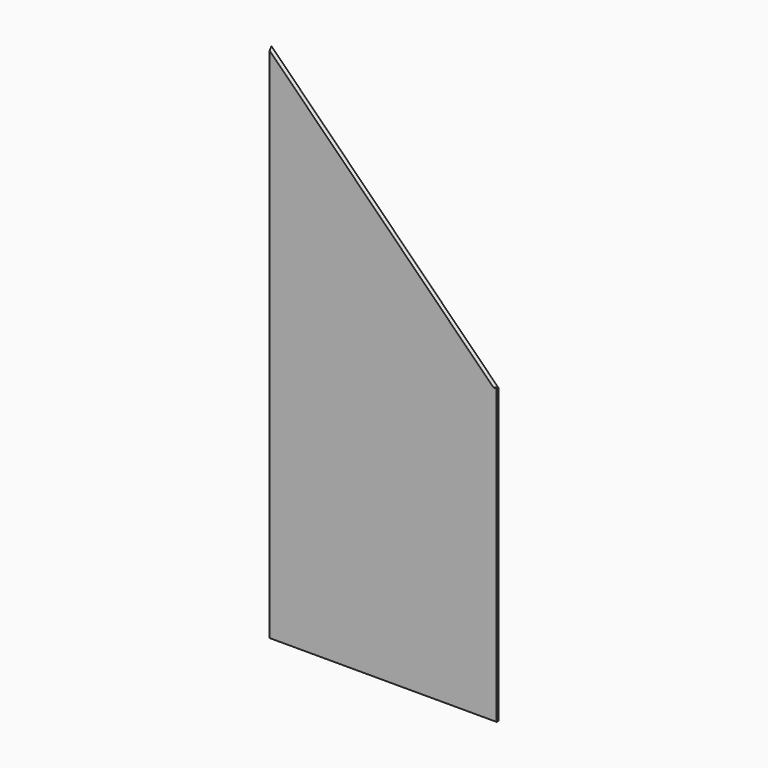
from build123d import *

# Parameters (mm, degrees)
F1_DEPTH = 4
F2_SIZE  = 3.99999
F4_DEPTH = 25


# Not quite as in the source:
# - a fillet or chamfer is up to 0.001 mm smaller than in the source, because OpenCascade refuses the exact size
# - ends of sketch curves that miss each other by under 0.0002 mm in the source are joined


with BuildPart() as f1:
    # F0 (on Front) → F1 (new body)
    with BuildSketch(Plane.XZ):
        Polygon((0, 944.56), (0, 0), (412.03, 0), (412.03, 532.53), align=None)
    extrude(amount=F1_DEPTH)

    # F2 (size 4 in the source; OpenCascade refuses exactly that, so slightly less here)
    f2_edges = [f1.edges().sort_by_distance(p)[0] for p in [
        (206.015, -4, 738.545),
    ]]
    chamfer(f2_edges, length=F2_SIZE)

    # F3 (on face) → F4 (join)
    with BuildSketch(Plane.YZ.offset(412.03)):
        Polygon((-4, 532.53), (-4, 526.8731457505), (-1e-05, 532.53), align=None)
    extrude(amount=-F4_DEPTH)


solid = f1.part
